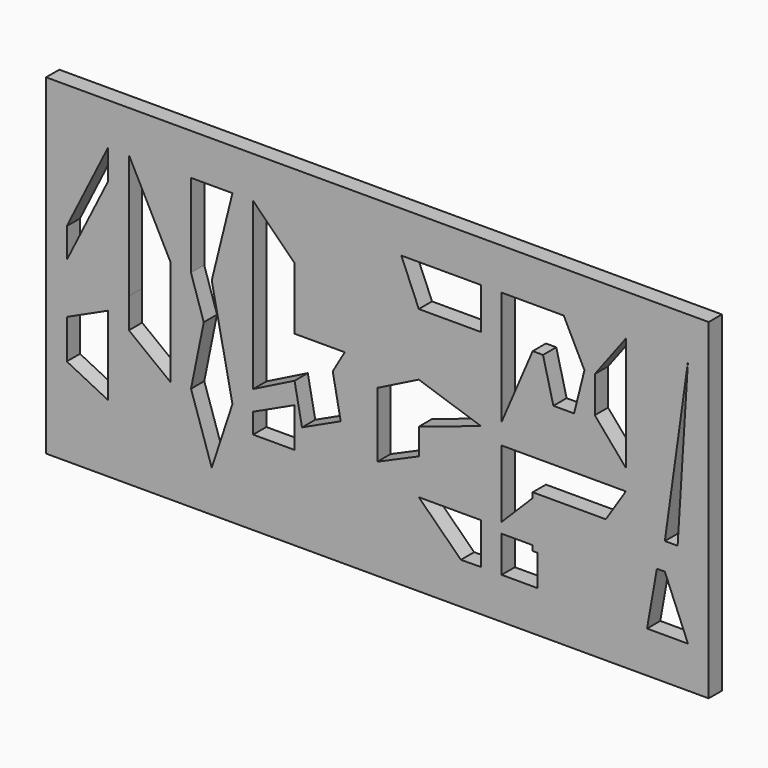
from build123d import *

# Parameters (mm, degrees)
F1_W     = 203.2
F1_H     = 101.6
F2_DEPTH = 5.08
F5_DEPTH = 25.4


with BuildPart() as f2:
    # F1 (on Front) → F2 (new body)
    with BuildSketch(Plane.XZ):
        with Locations((101.6, 50.8)):
            Rectangle(F1_W, F1_H)
    extrude(amount=-F2_DEPTH)

    # F4 (on face) → F5 (cut)
    with BuildSketch(Plane.XZ):
        Polygon((19.05, 88.9), (6.35, 63.4896950778), (6.35, 54.3535576701), (19.05, 79.7638625923), align=None)
        Polygon((19.05, 44.7899766155), (6.35, 38.9748217106), (6.35, 26.9433392146), (19.05, 20.5959144004), (19.05, 31.75), align=None)
        Polygon((25.4, 64.1602875233), (25.4, 50.8), (25.3980111729, 41.5485496718), (38.1, 31.75), (38.1, 50.8), (38.1, 64.1602875233), align=None)
        Polygon((25.4, 88.9), (25.4, 64.1602875233), (38.1, 64.1602875233), (38.1, 64.2026114812), align=None)
        Polygon((57.15, 88.9), (44.45, 88.9), (44.45, 63.2637151304), (48.3517487947, 51.1962487751), (44.45, 31.964471331), (50.8, 12.7), (57.15, 31.964471331), (53.2482512053, 51.1962487751), (50.8, 63.2637151304), align=None)
        Polygon((76.2, 76.2), (63.5, 88.9), (63.5, 38.0811007293), (76.2, 44.45), (78.4824932634, 32.6018280187), (90.3535660462, 38.1168511729), (87.9102185152, 50.8), (91.5801092576, 57.15), (76.2, 57.15), align=None)
        Polygon((76.2, 37.8645947099), (63.5, 31.964471331), (63.5, 25.7733563287), (76.2, 25.7733563287), align=None)
        Polygon((133.35, 50.8), (114.3, 57.15), (101.6, 50.8), (114.3, 44.45), align=None)
        Polygon((114.3, 44.45), (101.6, 50.8), (101.6, 30.8501303583), (114.3, 36.4221383274), align=None)
        Polygon((108.9507660084, 88.9), (114.3, 76.2), (133.35, 76.2), (133.35, 88.9), align=None)
        Polygon((133.35, 25.4), (114.3, 25.4), (127.2270479083, 12.7), (133.35, 12.7643318847), align=None)
        Polygon((149.225, 76.2), (152.4, 76.2), (158.75, 88.9), (139.7, 88.9), (139.7, 53.975), align=None)
        Polygon((158.75, 88.9), (152.4, 76.2), (155.575, 63.5), (161.925, 63.5), (165.1, 76.2), align=None)
        Polygon((177.8, 53.975), (177.8, 88.9), (168.275, 76.2), (168.275, 65.0875), align=None)
        Polygon((177.8, 47.625), (139.7, 47.625), (139.7, 26.9875), (149.225, 36.5125), (149.225, 38.1), (171.658446914, 38.1), align=None)
        Polygon((149.225, 23.8125), (139.7, 23.8125), (139.7, 12.7), (150.6915916045, 12.7), (150.6915916045, 22.225), (149.225, 22.225), align=None)
        Polygon((196.85, 88.9), (189.7574476064, 38.1), (193.675, 38.1), align=None)
        Polygon((196.85, 12.7), (189.7574476064, 29.845), (187.325, 29.845), (184.3011081219, 12.7), align=None)
    extrude(amount=-F5_DEPTH, mode=Mode.SUBTRACT)


solid = f2.part
